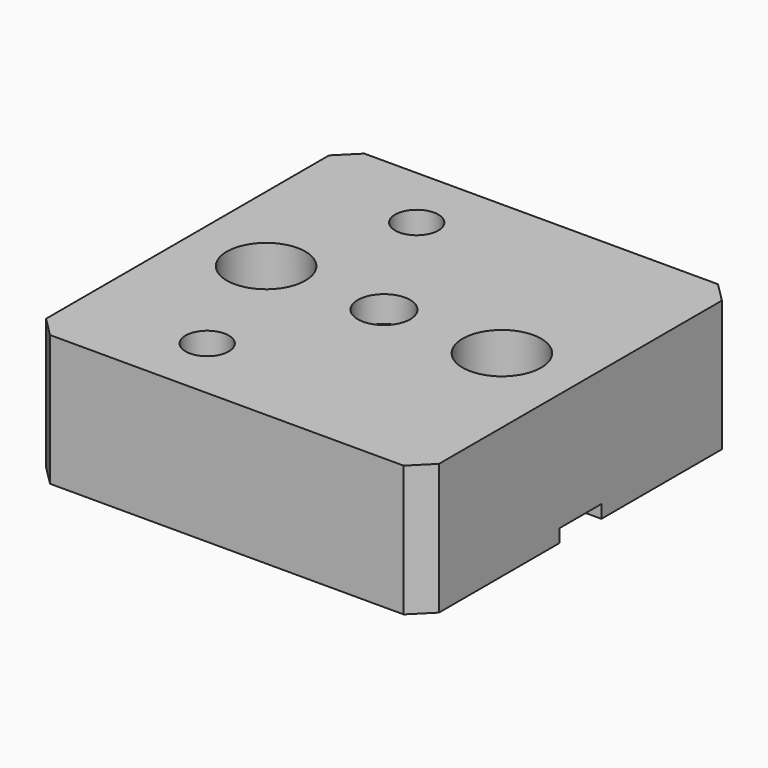
from build123d import *

# Parameters (mm, degrees)
F0_W     = 30
F0_H     = 30
F0_R     = 1.65
F0_R_2   = 3
F0_R_3   = 2
F0_R_4   = 1.5
F1_DEPTH = 10
F2_DEPTH = 12
F3_SIZE  = 1.5
F4_DEPTH = 4
F5_DEPTH = 8
F6_R     = 2
F7_DEPTH = 8
F6_R_2   = 1.5
F8_DEPTH = 1


# Not quite as in the source:
# - a feature names something its author has since deleted; it is built from what else it names


with BuildPart() as f1:
    # F0 (on Top) → F1 (new body)
    with BuildSketch(Plane.XY):
        with Locations((15, -15)):
            Rectangle(F0_W, F0_H)
        with Locations((9.5, -25)):
            Circle(F0_R, mode=Mode.SUBTRACT)
        with Locations((15, -24)):
            Circle(F0_R_2, mode=Mode.SUBTRACT)
        with Locations((6, -15)):
            Circle(F0_R_2, mode=Mode.SUBTRACT)
        with Locations((9.5, -5)):
            Circle(F0_R, mode=Mode.SUBTRACT)
        with Locations((15, -15)):
            Circle(F0_R_3, mode=Mode.SUBTRACT)
        with Locations((24, -15)):
            Circle(F0_R_2, mode=Mode.SUBTRACT)
        with Locations((15, -6)):
            Circle(F0_R_2, mode=Mode.SUBTRACT)
        with Locations((15, -15)):
            Circle(F0_R_3)
        with Locations((15, -6)):
            Circle(F0_R_2)
        with Locations((15, -6)):
            Circle(F0_R_4, mode=Mode.SUBTRACT)
        with Locations((15, -24)):
            Circle(F0_R_2)
        with Locations((15, -24)):
            Circle(F0_R_4, mode=Mode.SUBTRACT)
        with Locations((9.5, -5)):
            Circle(F0_R)
        with Locations((9.5, -25)):
            Circle(F0_R)
        with Locations((24, -15)):
            Circle(F0_R_2)
        with Locations((24, -15)):
            Circle(F0_R_4, mode=Mode.SUBTRACT)
        with Locations((6, -15)):
            Circle(F0_R_2)
        with Locations((6, -15)):
            Circle(F0_R_4, mode=Mode.SUBTRACT)
        with Locations((15, -24)):
            Circle(F0_R_4)
        with Locations((15, -6)):
            Circle(F0_R_4)
    extrude(amount=-F1_DEPTH)

    # F0 (on Top) → F2 (cut)
    with BuildSketch(Plane.XY):
        with Locations((15, -15)):
            Circle(F0_R_3)
    extrude(amount=-F2_DEPTH, mode=Mode.SUBTRACT)

    # F3
    f3_edges = [f1.edges().sort_by_distance(p)[0] for p in [
        (30, -30, -5),
        (0, -30, -5),
        (0, 0, -5),
        (30, 0, -5),
    ]]
    chamfer(f3_edges, length=F3_SIZE)

    # F0 (on Top) → F4 (cut)
    with BuildSketch(Plane.XY):
        with Locations((6, -15)):
            Circle(F0_R_2)
        with Locations((6, -15)):
            Circle(F0_R_4, mode=Mode.SUBTRACT)
        with Locations((24, -15)):
            Circle(F0_R_2)
        with Locations((24, -15)):
            Circle(F0_R_4, mode=Mode.SUBTRACT)
    extrude(amount=-F4_DEPTH, mode=Mode.SUBTRACT)

    # F0 (on Top) → F5 (cut)
    with BuildSketch(Plane.XY):
        with Locations((9.5, -5)):
            Circle(F0_R)
        with Locations((9.5, -25)):
            Circle(F0_R)
    extrude(amount=-F5_DEPTH, mode=Mode.SUBTRACT)

    # F6 (on face) → F7 (cut)
    with BuildSketch(Plane(origin=(0, 0, -10), x_dir=(1, 0, 0), z_dir=(0, 0, -1))):
        with BuildLine():
            ThreePointArc((19.6, 13.0404082058), (18, 15), (19.6, 16.9595917942))
            ThreePointArc((19.6, 16.9595917942), (10, 15), (19.6, 13.0404082058))
        make_face()
        with Locations((15, 15)):
            Circle(F6_R, mode=Mode.SUBTRACT)
        with BuildLine():
            ThreePointArc((19.6, 13.0404082058), (19.8989794856, 14), (20, 15))
            ThreePointArc((20, 15), (19.8989794856, 16), (19.6, 16.9595917942))
            ThreePointArc((19.6, 16.9595917942), (18, 15), (19.6, 13.0404082058))
        make_face()
    extrude(amount=-F7_DEPTH, mode=Mode.SUBTRACT)

    # F6 (on face) → F8 (cut)
    with BuildSketch(Plane(origin=(0, 0, -10), x_dir=(1, 0, 0), z_dir=(0, 0, -1))):
        with BuildLine():
            ThreePointArc((19.6, 16.9595917942), (19.8989794856, 16), (20, 15))
            ThreePointArc((20, 15), (19.8989794856, 14), (19.6, 13.0404082058))
            ThreePointArc((19.6, 13.0404082058), (19.798982076, 13.010127694), (20, 13))
            Line((20, 13), (30, 13))
            Line((30, 13), (30, 17))
            Line((30, 17), (20, 17))
            ThreePointArc((20, 17), (19.798982076, 16.989872306), (19.6, 16.9595917942))
        make_face()
        with Locations((24, 15)):
            Circle(F6_R_2, mode=Mode.SUBTRACT)
    extrude(amount=-F8_DEPTH, mode=Mode.SUBTRACT)


solid = f1.part
